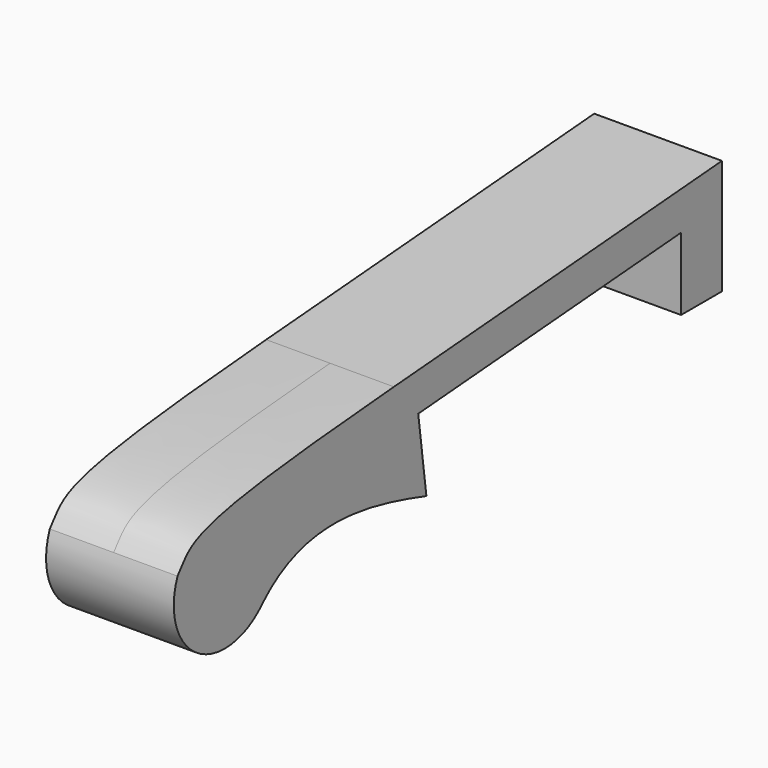
from build123d import *

# Parameters (mm, degrees)
F1_DEPTH = 25


# Not quite as in the source:
# - a feature of the source that left no trace in its solid (it failed there, or was rolled back) is left out


with BuildPart() as f1:
    # F0 (on Right) → F1 (new body, symmetric)
    with BuildSketch(Plane.YZ):
        with BuildLine():
            Line((-10, 28.3795828863), (-10, 0))
            Line((-10, 0), (10, 0))
            Line((10, 0), (10, 45))
            Line((10, 45), (-150.503690731, 32.3680855878))
            add(Edge.make_bspline(
                [(-150.503690731, 32.3680855878), (-251.6470152481, 24.4079333144), (-248.2635080814, 20.058169961), (-256.3765901785, 10.171615941)],
                knots=[0, 0, 0, 0, 108.1746463003, 108.1746463003, 108.1746463003, 108.1746463003], degree=3))
            ThreePointArc((-256.3765901785, 10.171615941), (-246.5433476591, -20.3637900829), (-214.7508155307, -16.0814332135))
            add(Edge.make_bspline(
                [(-214.7508155307, -16.0814332135), (-193.5426698765, 4.8777479678), (-161.3064821603, -3.4644254483), (-134.6062239053, -11.7416404626)],
                knots=[0, 0, 0, 0, 80.2620045097, 80.2620045097, 80.2620045097, 80.2620045097], degree=3))
            Line((-134.6062239053, -11.7416404626), (-138.6023360516, 18.2583595374))
            Line((-138.6023360516, 18.2583595374), (-10, 28.3795828863))
        make_face()
    extrude(amount=F1_DEPTH, both=True)


solid = f1.part
